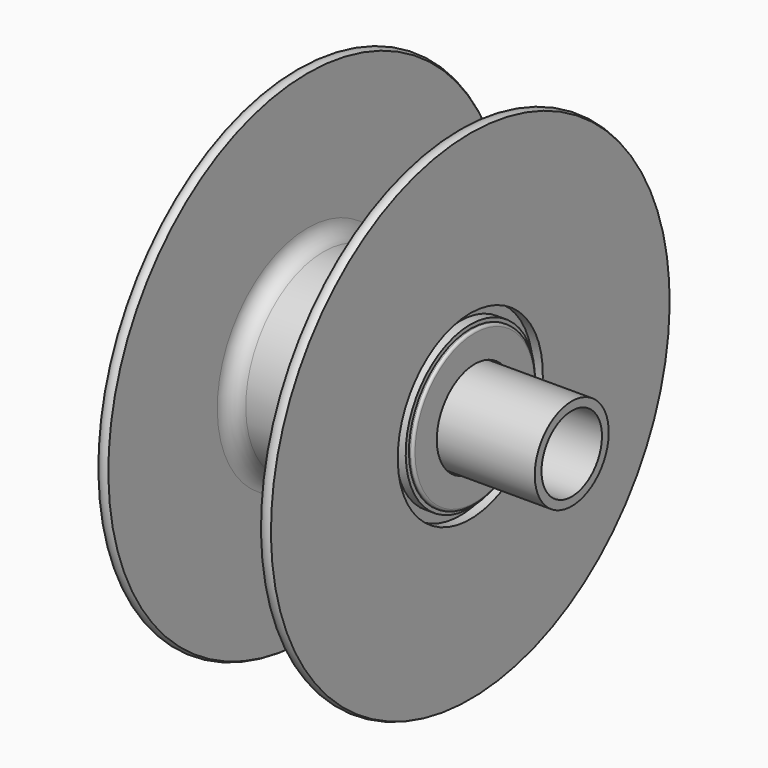
from build123d import *

# Parameters (mm, degrees)
F0_W   = 151.9453898072
F0_H   = 3.3889357001
F2_R   = 1
F2_2_R = 1


# Not quite as in the source:
# - a feature names something its author has since deleted; it is built from what else it names


with BuildPart() as f1:
    # F0 (on Front) → F1 (revolve)
    with BuildSketch(Plane.XZ):
        with BuildLine():
            Line((-34.1884475201, 29.4), (-0.0061754836, 29.4))
            Line((-0.0061754836, 29.4), (35.0615524799, 29.4))
            Line((35.0615524799, 29.4), (35.0615524799, 32.4))
            Line((35.0615524799, 32.4), (31.0615524799, 32.4))
            Line((31.0615524799, 32.4), (31.0615524799, 36.4))
            Line((31.0615524799, 36.4), (35.0615524799, 36.4))
            Line((35.0615524799, 36.4), (35.0615524799, 100))
            ThreePointArc((35.0615524799, 100), (33.0615524799, 100.5382707476), (31.0615524799, 100))
            Line((31.0615524799, 100), (31.0615524799, 45.35))
            ThreePointArc((31.0615524799, 45.35), (29.2016805404, 40.8598719395), (24.7115524799, 39))
            Line((24.7115524799, 39), (-23.8384475201, 39))
            ThreePointArc((-23.8384475201, 39), (-28.3285755807, 40.8598719395), (-30.1884475201, 45.35))
            Line((-30.1884475201, 45.35), (-30.1884475201, 100))
            ThreePointArc((-30.1884475201, 100), (-32.1884475201, 100.7606116789), (-34.1884475201, 100))
            Line((-34.1884475201, 100), (-34.1884475201, 36.4))
            Line((-34.1884475201, 36.4), (-30.1884475201, 36.4))
            Line((-30.1884475201, 36.4), (-30.1884475201, 32.4))
            Line((-30.1884475201, 32.4), (-34.1884475201, 32.4))
            Line((-34.1884475201, 32.4), (-34.1884475201, 29.4))
        make_face()
    revolve(axis=Axis((0.6704887888, 0, 0), (1, 0, 0)))


with BuildPart() as f1b:
    # F0 (on Front) → F1, piece 2 (revolve)
    with BuildSketch(Plane.XZ):
        Polygon((-36.3245010376, 19.05), (-30.1989875734, 19.05), (-30.1989875734, 29.2310900986), (-34.3979224563, 29.2310900986), (-34.3979224563, 30.9), (-36.3245010376, 30.9), align=None)
    revolve(axis=Axis((0.6704887888, 0, 0), (1, 0, 0)))

    # F2#2
    f2_2_edges = [f1b.edges().sort_by_distance(p)[0] for p in [
        (-36.324501, 0, -30.9),
    ]]
    fillet(f2_2_edges, radius=F2_2_R)


with BuildPart() as f1c:
    # F0 (on Front) → F1, piece 3 (revolve)
    with BuildSketch(Plane.XZ):
        Polygon((31.0908566462, 29.2185264379), (31.0908566462, 19.05), (36.8601419032, 19.05), (36.8601419032, 30.9599618167), (35.23087129, 30.9599618167), (35.23087129, 29.2185264379), align=None)
    revolve(axis=Axis((0.6704887888, 0, 0), (1, 0, 0)))

    # F2
    f2_edges = [f1c.edges().sort_by_distance(p)[0] for p in [
        (36.860142, 0, -30.959962),
    ]]
    fillet(f2_edges, radius=F2_R)


with BuildPart() as f1d:
    # F0 (on Front) → F1, piece 4 (revolve)
    with BuildSketch(Plane.XZ):
        with Locations((-0.1975260675, 16.8599756435)):
            Rectangle(F0_W, F0_H)
    revolve(axis=Axis((0.6704887888, 0, 0), (1, 0, 0)))


solid = Compound([f1.part, f1b.part, f1c.part, f1d.part])
